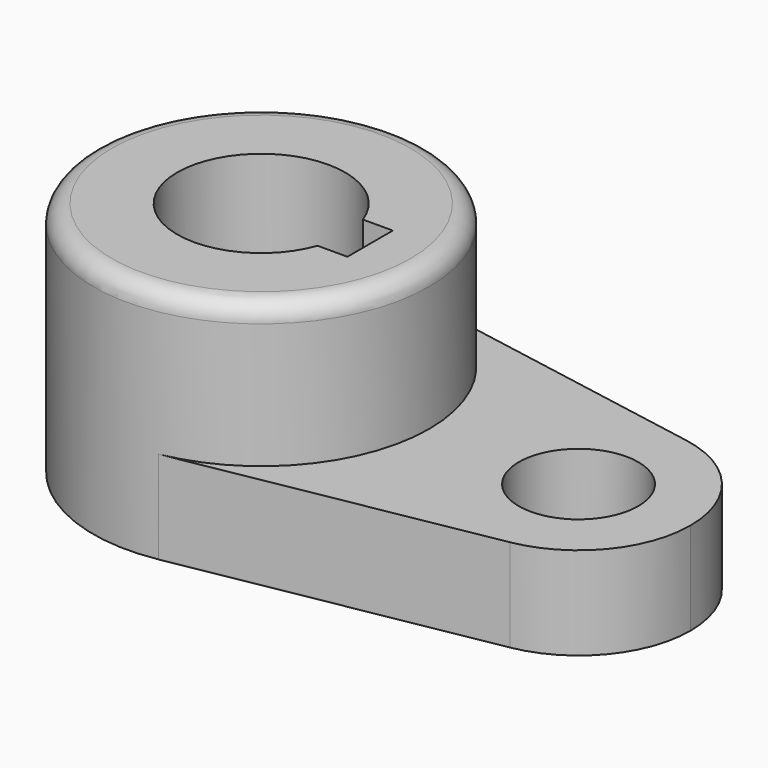
from build123d import *

# Parameters (mm, degrees)
F0_R     = 10.16
F1_DEPTH = 15.76169
F2_DEPTH = 40.2358
F3_R     = 3.175


# Not quite as in the source:
# - a feature names something its author has since deleted; it is built from what else it names


with BuildPart() as f1:
    # F0 (on Top) → F1 (new body)
    with BuildSketch(Plane.XY):
        with BuildLine():
            ThreePointArc((5.0426470588, -28.1265414802), (21.9160245563, -18.3362616868), (28.575, 0))
            ThreePointArc((28.575, 0), (21.9160245563, 18.3362616868), (5.0426470588, 28.1265414802))
            ThreePointArc((5.0426470588, 28.1265414802), (-28.575, 0), (5.0426470588, -28.1265414802))
        make_face()
        with BuildLine():
            ThreePointArc((-13.4477648793, 4.826), (0, 14.2875), (13.4477648793, 4.826))
            Line((13.4477648793, 4.826), (18.5277648793, 4.826))
            Line((18.5277648793, 4.826), (18.5277648793, -4.826))
            Line((18.5277648793, -4.826), (13.4477648793, -4.826))
            ThreePointArc((13.4477648793, -4.826), (0, -14.2875), (-13.4477648793, -4.826))
            Line((-13.4477648793, -4.826), (-18.5277648793, -4.826))
            Line((-18.5277648793, -4.826), (-18.5277648793, 4.826))
            Line((-18.5277648793, 4.826), (-13.4477648793, 4.826))
        make_face(mode=Mode.SUBTRACT)
        with BuildLine():
            ThreePointArc((5.0426470588, 28.1265414802), (21.9160245563, 18.3362616868), (28.575, 0))
            ThreePointArc((28.575, 0), (21.9160245563, -18.3362616868), (5.0426470588, -28.1265414802))
            Line((5.0426470588, -28.1265414802), (57.3367647059, -18.7510276535))
            ThreePointArc((57.3367647059, -18.7510276535), (34.925, 0), (57.3367647059, 18.7510276535))
            Line((57.3367647059, 18.7510276535), (5.0426470588, 28.1265414802))
        make_face()
        with BuildLine():
            ThreePointArc((-13.4477648793, -4.826), (-14.2875, 0), (-13.4477648793, 4.826))
            Line((-13.4477648793, 4.826), (-18.5277648793, 4.826))
            Line((-18.5277648793, 4.826), (-18.5277648793, -4.826))
            Line((-18.5277648793, -4.826), (-13.4477648793, -4.826))
        make_face()
        with BuildLine():
            ThreePointArc((73.025, 0), (68.5856830375, 12.2241744579), (57.3367647059, 18.7510276535))
            ThreePointArc((57.3367647059, 18.7510276535), (34.925, 0), (57.3367647059, -18.7510276535))
            ThreePointArc((57.3367647059, -18.7510276535), (68.5856830375, -12.2241744579), (73.025, 0))
        make_face()
        with Locations((53.975, 0)):
            Circle(F0_R, mode=Mode.SUBTRACT)
    extrude(amount=F1_DEPTH)

    # F0 (on Top) → F2 (join)
    with BuildSketch(Plane.XY):
        with BuildLine():
            ThreePointArc((5.0426470588, -28.1265414802), (21.9160245563, -18.3362616868), (28.575, 0))
            ThreePointArc((28.575, 0), (21.9160245563, 18.3362616868), (5.0426470588, 28.1265414802))
            ThreePointArc((5.0426470588, 28.1265414802), (-28.575, 0), (5.0426470588, -28.1265414802))
        make_face()
        with BuildLine():
            ThreePointArc((-13.4477648793, 4.826), (0, 14.2875), (13.4477648793, 4.826))
            Line((13.4477648793, 4.826), (18.5277648793, 4.826))
            Line((18.5277648793, 4.826), (18.5277648793, -4.826))
            Line((18.5277648793, -4.826), (13.4477648793, -4.826))
            ThreePointArc((13.4477648793, -4.826), (0, -14.2875), (-13.4477648793, -4.826))
            Line((-13.4477648793, -4.826), (-18.5277648793, -4.826))
            Line((-18.5277648793, -4.826), (-18.5277648793, 4.826))
            Line((-18.5277648793, 4.826), (-13.4477648793, 4.826))
        make_face(mode=Mode.SUBTRACT)
        with BuildLine():
            ThreePointArc((-13.4477648793, -4.826), (-14.2875, 0), (-13.4477648793, 4.826))
            Line((-13.4477648793, 4.826), (-18.5277648793, 4.826))
            Line((-18.5277648793, 4.826), (-18.5277648793, -4.826))
            Line((-18.5277648793, -4.826), (-13.4477648793, -4.826))
        make_face()
    extrude(amount=F2_DEPTH)

    # F3
    f3_edges = [f1.edges().sort_by_distance(p)[0] for p in [
        (-5.042647, 28.126541, 40.2358),
    ]]
    fillet(f3_edges, radius=F3_R)


solid = f1.part
